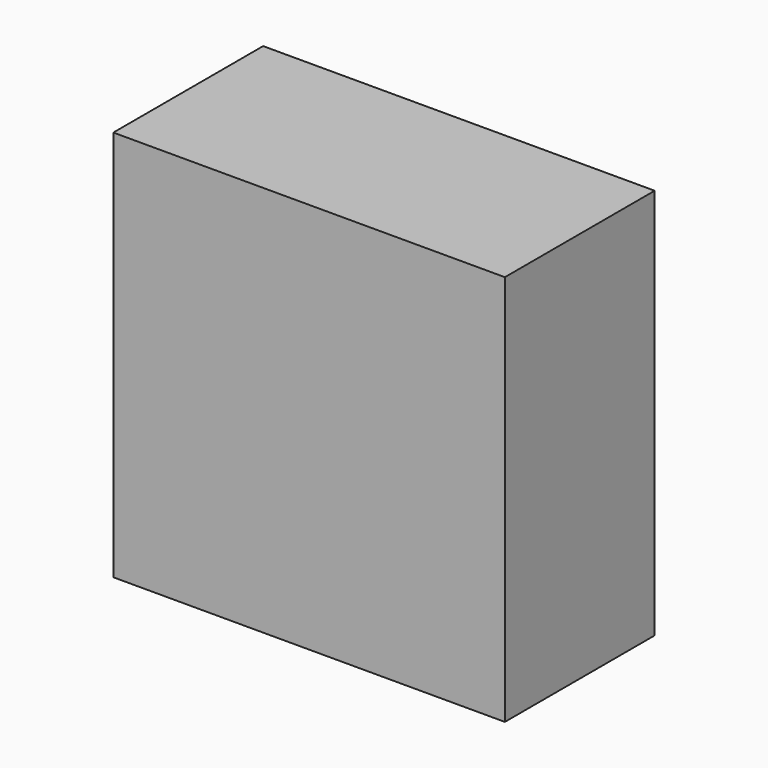
from build123d import *

# Parameters (mm, degrees)
F0_W     = 31.8670235574
F0_H     = 31.8670235574
F2_DEPTH = 15.24


# Not quite as in the source:
# - the program builds the solid bodies; features that only make, move or delete a surface that nothing else refers to are left out


with BuildPart() as f2:
    # F0 (on Front) → F2 (new body)
    with BuildSketch(Plane.XZ):
        with Locations((-15.9335117787, 21.2193038315)):
            Rectangle(F0_W, F0_H)
    extrude(amount=F2_DEPTH)


solid = f2.part
